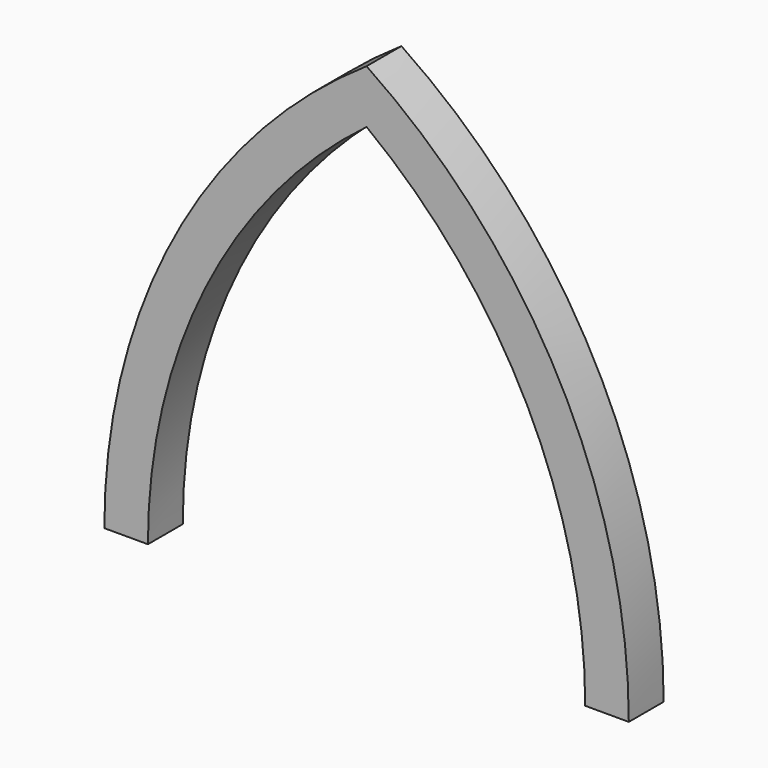
from build123d import *

# Parameters (mm, degrees)
F1_DEPTH = 6.35


# Not quite as in the source:
# - ends of sketch curves that miss each other by under 0.0002 mm in the source are joined


with BuildPart() as f1:
    # F0 (on Front) → F1 (new body)
    with BuildSketch(Plane.XZ):
        with BuildLine():
            ThreePointArc((38.2175176824, 4.5037588412), (28.0665538033, 45.1268115764), (0, 76.2))
            ThreePointArc((0, 76.2), (-28.0665538033, 45.1268115764), (-38.2175176824, 4.5037588412))
            Line((-38.2175176824, 4.5037588412), (-31.8675123234, 4.5037588412))
            ThreePointArc((-31.8675123234, 4.5037588412), (-23.4587753486, 40.2089414997), (0, 68.4091699138))
            ThreePointArc((0, 68.4091699138), (23.4587753486, 40.2089414997), (31.8675181077, 4.5037588412))
            Line((31.8675181077, 4.5037588412), (38.2175176824, 4.5037588412))
        make_face()
    extrude(amount=F1_DEPTH)


solid = f1.part
